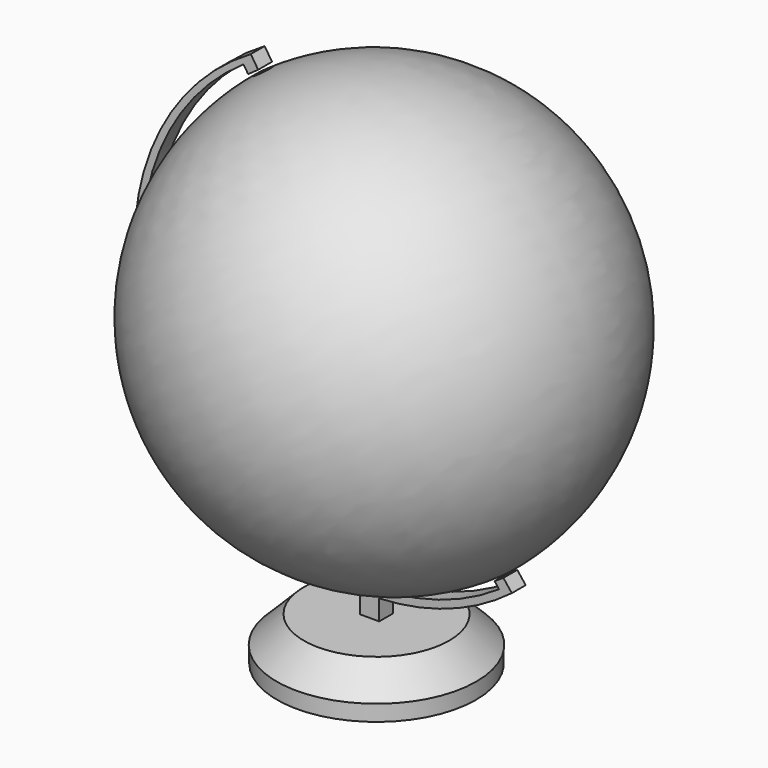
from build123d import *

# Parameters (mm, degrees)
F7_DEPTH      = 3.81
F7_DEPTH_BACK = 3.81
F8_R          = 57.3128960448
F8_W          = 8.4502474715
F8_H          = 7.62
F9_DEPTH      = 11.938
F11_R         = 43.6922740834
F11_W         = 8.4502474715
F11_H         = 7.62
F12_DEPTH     = 7.112


# Not quite as in the source:
# - a fillet or chamfer that OpenCascade refuses, or shapes differently, is made with other operations: its cross-section is extruded or revolved along the edge and cut away or added
# - the program builds the solid bodies; features that only make, move or delete a surface that nothing else refers to are left out


with BuildPart() as f5:
    # F4 (on Front) → F5 (revolve)
    with BuildSketch(Plane.XZ):
        with BuildLine():
            ThreePointArc((58.8755346835, -72.158806026), (79.0942790348, 56.5321782393), (-47.4915131927, 87.292611599))
            Line((-47.4915131927, 87.292611599), (58.8755346835, -72.158806026))
        make_face()
    revolve(axis=Axis((2.4909305948, 0, 5.4456610979), (0.5549389309, 0, -0.8318910884)))


with BuildPart() as f7:
    # F6 (on Front) → F7 (new body, two sides)
    with BuildSketch(Plane.XZ) as f7_sk:
        with BuildLine():
            Line((-54.1473962367, 84.5184549689), (-49.7353225946, 87.6264721155))
            Line((-49.7353225946, 87.6264721155), (-52.9789444648, 92.6372483192))
            ThreePointArc((-52.9789444648, 92.6372483192), (-100.9016267075, -21.3708152974), (-5.0204185613, -99.4810961019))
            Line((-5.0204185613, -99.4810961019), (3.4298289102, -99.4810961019))
            Line((3.4298289102, -99.4810961019), (3.4298289102, -99.4819933614))
            ThreePointArc((3.4298289102, -99.4819933614), (34.161363591, -93.4706552038), (61.6748090034, -78.5182730584))
            Line((61.6748090034, -78.5182730584), (57.9917654395, -73.8074108958))
            Line((57.9917654395, -73.8074108958), (54.1345439851, -76.3141438365))
            Line((54.1345439851, -76.3141438365), (56.0401518351, -78.8536878354))
            ThreePointArc((56.0401518351, -78.8536878354), (-83.3037308216, -51.7174105412), (-56.1674535275, 87.6264721155))
            Line((-56.1674535275, 87.6264721155), (-54.4421227455, 84.9611656242))
            Line((-54.4421227455, 84.9611656242), (-54.1473962367, 84.5184549689))
        make_face()
    extrude(amount=F7_DEPTH)
    extrude(f7_sk.sketch, amount=-F7_DEPTH_BACK)


with BuildPart() as f7b:
    # F6 (on Front) → F7, piece 2 (new body, two sides)
    with BuildSketch(Plane.XZ) as f7_2_sk:
        with BuildLine():
            ThreePointArc((3.4298289102, -99.4819933614), (-0.7953040141, -99.5680804241), (-5.0204185613, -99.4810961019))
            Line((-5.0204185613, -99.4810961019), (-5.0204185613, -108.3873957396))
            Line((-5.0204185613, -108.3873957396), (3.4298289102, -108.3873957396))
            Line((3.4298289102, -108.3873957396), (3.4298289102, -99.4819933614))
        make_face()
    extrude(amount=F7_DEPTH)
    extrude(f7_2_sk.sketch, amount=-F7_DEPTH_BACK)


with BuildPart() as f9:
    # F8 (on face) → F9 (new body)
    with BuildSketch(Plane(origin=(0, 0, -108.3873957396), x_dir=(1, 0, 0), z_dir=(0, 0, -1))):
        with Locations((-0.7952948256, 0)):
            Circle(F8_R)
        with Locations((-0.7952948256, 0)):
            Rectangle(F8_W, F8_H, mode=Mode.SUBTRACT)
    extrude(amount=F9_DEPTH)

    # F10: chamfer of 25.4 on 1 edges, made by hand

    # F10_s1 → F10_t2 (revolve, cut)
    with BuildSketch(Plane.XZ):
        Polygon((56.5176012193, -133.7873957396), (31.1176012193, -108.3873957396), (56.5176012193, -108.3873957396), align=None)
    revolve(axis=Axis((-0.7952948256, 0, -108.3873957396), (0, 0, -1)), mode=Mode.SUBTRACT)

    # F11 (on face) → F12 (join)
    with BuildSketch(Plane(origin=(0, 0, -120.3253957396), x_dir=(1, 0, 0), z_dir=(0, 0, -1))):
        with Locations((-0.7952948256, 0)):
            Circle(F11_R)
        with Locations((-0.7952948256, 0)):
            Rectangle(F11_W, F11_H, mode=Mode.SUBTRACT)
    extrude(amount=F12_DEPTH)


solid = Compound([f5.part, f7.part, f7b.part, f9.part])
